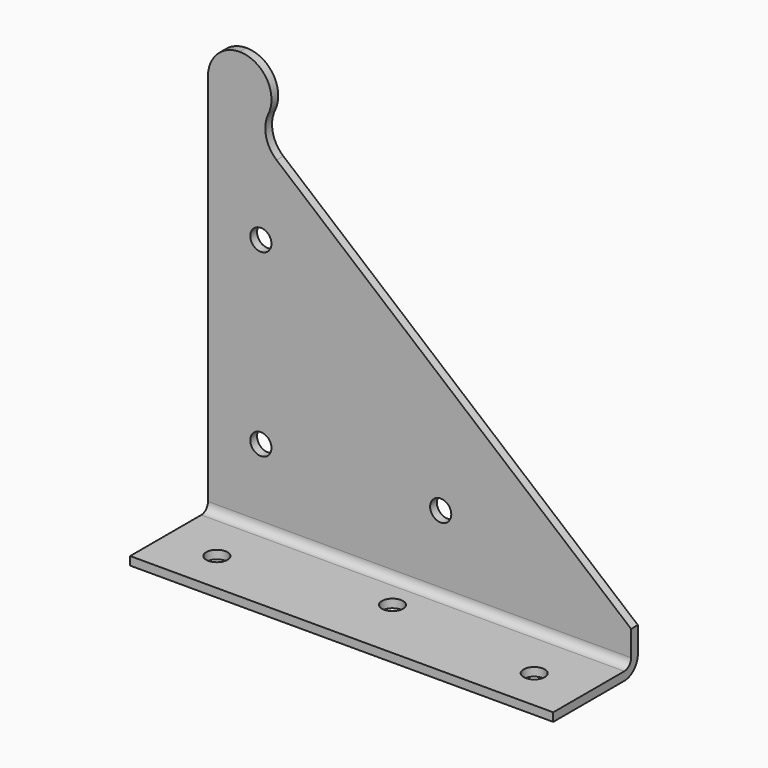
from build123d import *

# Parameters (mm, degrees)
F1_DEPTH = 100
F3_DEPTH = 4.001
F4_R     = 5
F5_DEPTH = 4.001
F6_R     = 5
F7_DEPTH = 4.001


# Not quite as in the source:
# - a feature names something its author has since deleted; it is built from what else it names


with BuildPart() as f1:
    # F0 (on Right) → F1 (new body, symmetric)
    with BuildSketch(Plane.YZ):
        with BuildLine():
            Line((0, 192), (0, 0))
            ThreePointArc((0, 0), (-1.1715728753, -2.8284271247), (-4, -4))
            Line((-4, -4), (-46, -4))
            Line((-46, -4), (-46, -8))
            Line((-46, -8), (-4, -8))
            ThreePointArc((-4, -8), (1.6568542495, -5.6568542495), (4, 0))
            Line((4, 0), (4, 192))
            Line((4, 192), (0, 192))
        make_face()
    extrude(amount=F1_DEPTH, both=True)

    # F2 (on face) → F3 (cut, through all)
    with BuildSketch(Plane.XZ):
        with BuildLine():
            Line((-67.5611548883, 152.6005032665), (100, 12))
            Line((100, 12), (100, 192))
            Line((100, 192), (-85, 192))
            ThreePointArc((-85, 192), (-72.3150438383, 185.0057408886), (-71.4596703715, 170.5455849566))
            ThreePointArc((-71.4596703715, 170.5455849566), (-72.5774250894, 160.9067448009), (-67.5611548883, 152.6005032665))
        make_face()
        with BuildLine():
            ThreePointArc((-100, 177), (-95.6066017178, 187.6066017178), (-85, 192))
            Line((-85, 192), (-100, 192))
            Line((-100, 192), (-100, 177))
        make_face()
    extrude(amount=-F3_DEPTH, mode=Mode.SUBTRACT)

    # F4 (on face) → F5 (cut, through all)
    with BuildSketch(Plane.XZ):
        with Locations((-75, 32)):
            Circle(F4_R)
        with Locations((10, 32)):
            Circle(F4_R)
        with Locations((-75, 117)):
            Circle(F4_R)
    extrude(amount=-F5_DEPTH, mode=Mode.SUBTRACT)

    # F6 (on face) → F7 (cut, through all)
    with BuildSketch(Plane.XY.offset(-4)):
        with Locations((-75, -26)):
            Circle(F6_R)
        with Locations((0, -16)):
            Circle(F6_R)
        with Locations((75, -26)):
            Circle(F6_R)
    extrude(amount=-F7_DEPTH, mode=Mode.SUBTRACT)


solid = f1.part
